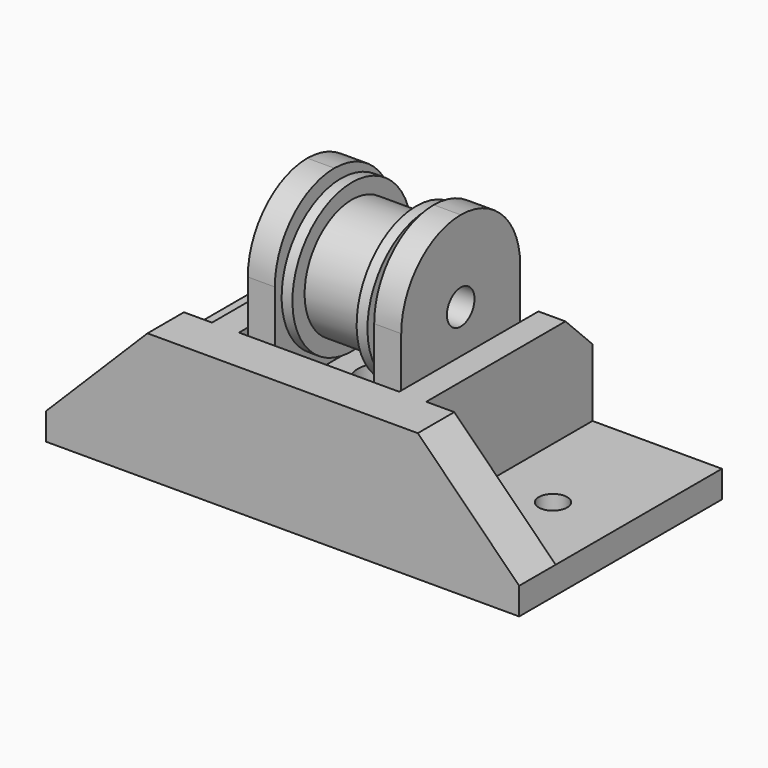
from build123d import *

# Parameters (mm, degrees)
F3_R      = 7.987
F4_DEPTH  = 4.8
F5_R      = 7.987
F6_DEPTH  = 4.8
F2_R      = 2.5
F7_DEPTH  = 12.701
F10_DEPTH = 22
F11_R     = 2.55
F12_DEPTH = 22.701
F13_R     = 10.99999
F14_R     = 2.15
F15_DEPTH = 8
F16_R     = 3.875
F17_DEPTH = 4.5
F18_W     = 70
F18_H     = 37.5
F19_DEPTH = 4
F20_W     = 4
F20_H     = 37.5
F21_DEPTH = 15
F22_W     = 70
F22_H     = 6.75
F23_DEPTH = 15
F24_SIZE  = 15
F25_SIZE  = 5
F26_R     = 2.15
F27_DEPTH = 4
F28_R     = 2.1
F29_DEPTH = 4


# Not quite as in the source:
# - a fillet or chamfer is up to 0.001 mm smaller than in the source, because OpenCascade refuses the exact size


with BuildPart() as f1:
    # F0 (on Front) → F1 (revolve)
    with BuildSketch(Plane.XZ):
        Polygon((-6.35, 11), (-6.35, 0), (6.35, 0), (6.35, 11), (4.75, 11), (4.75, 8.75), (0, 8.75), (-4.75, 8.75), (-4.75, 11), align=None)
    revolve(axis=Axis((1.279097545, 0, 0), (1, 0, 0)))

    # F3 (on face) → F4 (cut)
    with BuildSketch(Plane(origin=(-6.35, 0, 0), x_dir=(0, -1, 0), z_dir=(-1, 0, 0))):
        Circle(F3_R)
    extrude(amount=-F4_DEPTH, mode=Mode.SUBTRACT)

    # F5 (on face) → F6 (cut)
    with BuildSketch(Plane.YZ.offset(6.35)):
        Circle(F5_R)
    extrude(amount=-F6_DEPTH, mode=Mode.SUBTRACT)

    # F2 (on face) → F7 (cut, through all)
    with BuildSketch(Plane(origin=(-6.35, 0, 0), x_dir=(0, -1, 0), z_dir=(-1, 0, 0))):
        Circle(F2_R)
    extrude(amount=-F7_DEPTH, mode=Mode.SUBTRACT)


with BuildPart() as f10:
    # F9 (on offset) → F10 (new body)
    with BuildSketch(Plane.XZ.offset(11)):
        Polygon((7.35, 12), (7.35, 0), (7.35, -13), (0, -13), (-7.35, -13), (-7.35, 0), (-7.35, 12), (-11.35, 12), (-11.35, -21), (0, -21), (11.35, -21), (11.35, 12), align=None)
    extrude(amount=-F10_DEPTH)

    # F11 (on face) → F12 (cut, through all)
    with BuildSketch(Plane.YZ.offset(11.35)):
        Circle(F11_R)
    extrude(amount=-F12_DEPTH, mode=Mode.SUBTRACT)

    # F13 (radius 11 in the source; OpenCascade refuses exactly that, so slightly less here)
    f13_edges = [f10.edges().sort_by_distance(p)[0] for p in [
        (-9.35, 11, 12),
        (9.35, 11, 12),
        (-9.35, -11, 12),
        (9.35, -11, 12),
    ]]
    fillet(f13_edges, radius=F13_R)

    # F14 (on face) → F15 (cut, through all)
    with BuildSketch(Plane(origin=(0, 0, -21), x_dir=(1, 0, 0), z_dir=(0, 0, -1))):
        Circle(F14_R)
    extrude(amount=-F15_DEPTH, mode=Mode.SUBTRACT)

    # F16 (on face) → F17 (cut)
    with BuildSketch(Plane.XY.offset(-13)):
        Circle(F16_R)
    extrude(amount=-F17_DEPTH, mode=Mode.SUBTRACT)


with BuildPart() as f19:
    # F18 (on face) → F19 (new body)
    with BuildSketch(Plane(origin=(0, 0, -21), x_dir=(1, 0, 0), z_dir=(0, 0, -1))):
        Rectangle(F18_W, F18_H)
    extrude(amount=F19_DEPTH)

    # F20 (on face) → F21 (join)
    with BuildSketch(Plane.XY.offset(-21)):
        with Locations((-13.85, 0)):
            Rectangle(F20_W, F20_H)
        with Locations((13.85, 0)):
            Rectangle(F20_W, F20_H)
    extrude(amount=F21_DEPTH)

    # F22 (on face) → F23 (join, through all)
    with BuildSketch(Plane.XY.offset(-21)):
        with Locations((0, -15.375)):
            Rectangle(F22_W, F22_H)
    extrude(amount=F23_DEPTH)

    # F24
    f24_edges = [f19.edges().sort_by_distance(p)[0] for p in [
        (35, -15.375, -6),
        (-35, -15.375, -6),
    ]]
    chamfer(f24_edges, length=F24_SIZE)

    # F25
    f25_edges = [f19.edges().sort_by_distance(p)[0] for p in [
        (-13.85, 18.75, -6),
        (13.85, 18.75, -6),
    ]]
    chamfer(f25_edges, length=F25_SIZE)

    # F26 (on face) → F27 (cut, through all)
    with BuildSketch(Plane(origin=(0, 0, -25), x_dir=(1, 0, 0), z_dir=(0, 0, -1))):
        Circle(F26_R)
    extrude(amount=-F27_DEPTH, mode=Mode.SUBTRACT)

    # F28 (on face) → F29 (cut, through all)
    with BuildSketch(Plane(origin=(0, 0, -25), x_dir=(1, 0, 0), z_dir=(0, 0, -1))):
        with Locations((-25, 0)):
            Circle(F28_R)
        with Locations((25, 0)):
            Circle(F28_R)
    extrude(amount=-F29_DEPTH, mode=Mode.SUBTRACT)


solid = Compound([f1.part, f10.part, f19.part])
